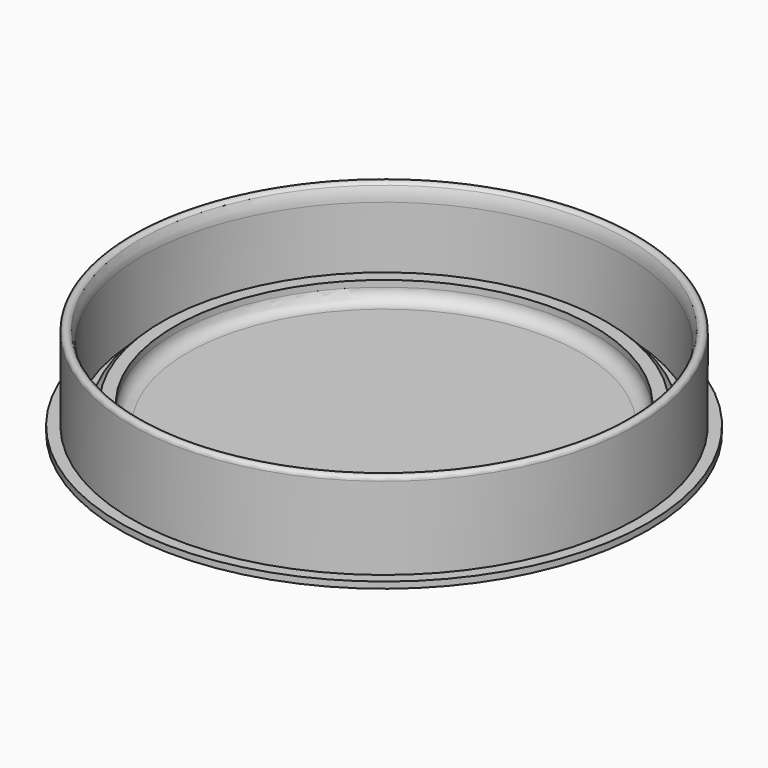
from build123d import *

# Parameters (mm, degrees)
F0_R     = 41.5
F1_DEPTH = 1
F2_R     = 39.75
F2_R_2   = 37.95
F3_DEPTH = 15
F4_R     = 35.95
F4_R_2   = 32.95
F5_DEPTH = 3
F6_SIZE  = 1
F8_R     = 0.7
F9_R     = 2


# Not quite as in the source:
# - a fillet or chamfer that OpenCascade refuses, or shapes differently, is made with other operations: its cross-section is extruded or revolved along the edge and cut away or added


with BuildPart() as f1:
    # F0 (on Top) → F1 (new body)
    with BuildSketch(Plane.XY):
        Circle(F0_R)
    extrude(amount=F1_DEPTH)

    # F2 (on face) → F3 (join)
    with BuildSketch(Plane.XY.offset(1)):
        Circle(F2_R)
        Circle(F2_R_2, mode=Mode.SUBTRACT)
    extrude(amount=F3_DEPTH)

    # F4 (on face) → F5 (join)
    with BuildSketch(Plane.XY.offset(1)):
        Circle(F4_R)
        Circle(F4_R_2, mode=Mode.SUBTRACT)
    extrude(amount=F5_DEPTH)

    # F6
    f6_edges = [f1.edges().sort_by_distance(p)[0] for p in [
        (-35.95, 0, 4),
    ]]
    chamfer(f6_edges, length=F6_SIZE)

    # F7: fillet of radius 5 on 1 edges, made by hand

    # F7_s1 → F7_t2 (revolve, cut)
    with BuildSketch(Plane.XZ):
        with BuildLine():
            ThreePointArc((37.95, 12.1581254575), (38.4223074309, 14.2794458011), (39.75, 16))
            Line((39.75, 16), (37.95, 16))
            Line((37.95, 16), (37.95, 12.1581254575))
        make_face()
    revolve(axis=Axis((0, 0, 16), (0, 0, 1)), mode=Mode.SUBTRACT)

    # F8
    f8_edges = [f1.edges().sort_by_distance(p)[0] for p in [
        (-39.75, 0, 16),
    ]]
    fillet(f8_edges, radius=F8_R)

    # F9
    f9_edges = [f1.edges().sort_by_distance(p)[0] for p in [
        (-32.95, 0, 1),
    ]]
    fillet(f9_edges, radius=F9_R)


solid = f1.part
